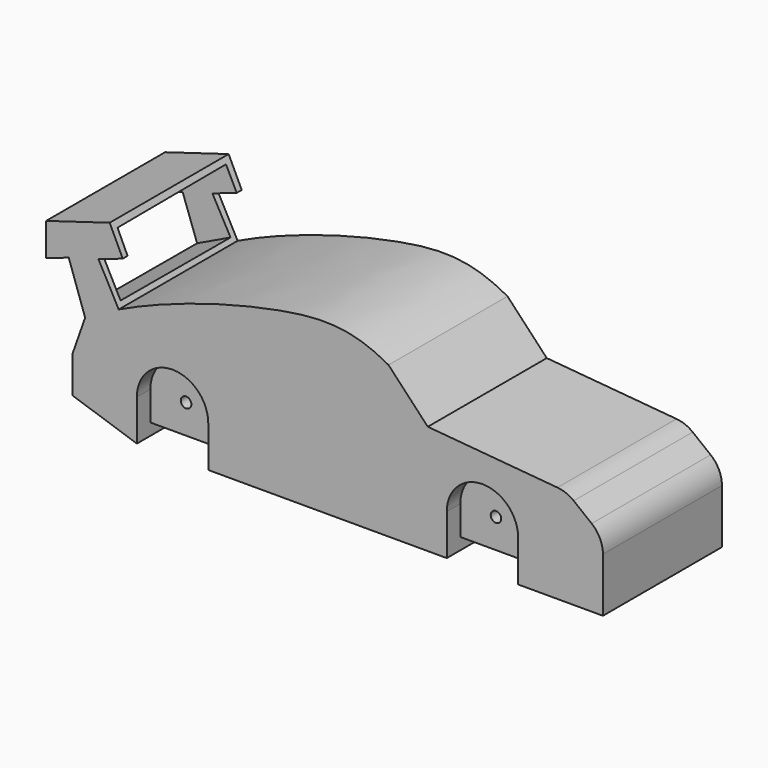
from build123d import *

# Parameters (mm, degrees)
F1_DEPTH  = 38.1
F3_DEPTH  = 25.4
F6_DEPTH  = 4.318
F8_DEPTH  = 4.318
F9_R      = 1.3609782851
F9_R_2    = 1.3503546706
F10_DEPTH = 61.214


# Not quite as in the source:
# - a feature names something its author has since deleted; it is built from what else it names


with BuildPart() as f1:
    # F0 (on Front) → F1 (new body)
    with BuildSketch(Plane.XZ):
        with BuildLine():
            Line((52.0340008008, 9.3591057662), (47.4384056476, 12.9927370075))
            ThreePointArc((47.4384056476, 12.9927370075), (45.4749605723, 14.1169814212), (43.2679541409, 14.615142718))
            Line((43.2679541409, 14.615142718), (10.0584002212, 17.5260007381))
            Line((10.0584002212, 17.5260007381), (0, 28.1940009445))
            add(Edge.make_bspline(
                [(0, 28.1940009445), (-9.1002955269, 33.2901659502), (-24.9064630473, 33.5549116559), (-55.7131559047, 24.6859865442), (-69.1292500573, 18.2258343206)],
                knots=[0, 0, 0, 0, 0.4163863711, 0.8919338321, 0.8919338321, 0.8919338321, 0.8919338321], degree=3))
            add(Edge.make_bspline(
                [(-69.1292500573, 18.2258343206), (-72.1780012369, 16.7577917973), (-75.0713687219, 15.2003305751), (-77.7240023017, 13.5635994375)],
                knots=[0.8919338321, 0.8919338321, 0.8919338321, 0.8919338321, 1, 1, 1, 1], degree=3))
            Line((-77.7240023017, 13.5635994375), (-80.9243991971, 4.4677392631))
            Line((-80.9243991971, 4.4677392631), (-80.9243991971, -5.0292001106))
            Line((-80.9243991971, -5.0292001106), (-64.465200973, -10.5156))
            Line((-64.465200973, -10.5156), (-64.465200973, -7.498764433))
            Line((-64.465200973, -7.498764433), (-64.465200973, 0))
            ThreePointArc((-64.465200973, 0), (-55.321200973, 9.144), (-46.177200973, 0))
            Line((-46.177200973, 0), (-46.177200973, -7.498764433))
            Line((-46.177200973, -7.498764433), (-46.177200973, -10.5156))
            Line((-46.177200973, -10.5156), (14.9299539626, -10.5156))
            Line((14.9299539626, -10.5156), (14.9299539626, -7.498764433))
            Line((14.9299539626, -7.498764433), (14.9299539626, 0))
            ThreePointArc((14.9299539626, 0), (24.076577276, 9.1466233134), (33.2232005894, 0))
            Line((33.2232005894, 0), (33.2232005894, -7.498764433))
            Line((33.2232005894, -7.498764433), (33.2232005894, -10.5156004429))
            Line((33.2232005894, -10.5156004429), (54.9278818071, -10.5156004429))
            Line((54.9278818071, -10.5156004429), (54.9278818071, 3.3817987423))
            ThreePointArc((54.9278818071, 3.3817987423), (54.1663592887, 6.7022936804), (52.0340008008, 9.3591057662))
        make_face()
        with BuildLine():
            add(Edge.make_bspline(
                [(-69.1292500573, 18.2258343206), (-72.1780012369, 16.7577917973), (-75.0713687219, 15.2003305751), (-77.7240023017, 13.5635994375)],
                knots=[0.8919338321, 0.8919338321, 0.8919338321, 0.8919338321, 1, 1, 1, 1], degree=3))
            Line((-69.1292500573, 18.2258343206), (-74.2949992421, 27.8891995555))
            Line((-74.2949992421, 27.8891995555), (-81.9149985909, 25.7555991411))
            Line((-81.9149985909, 25.7555991411), (-77.7240023017, 13.5635994375))
        make_face()
        with BuildLine():
            Line((14.9299539626, -7.498764433), (33.2232005894, -7.498764433))
            Line((33.2232005894, -7.498764433), (33.2232005894, 0))
            ThreePointArc((33.2232005894, 0), (24.076577276, 9.1466233134), (14.9299539626, 0))
            Line((14.9299539626, 0), (14.9299539626, -7.498764433))
        make_face()
        Polygon((-81.9149985909, 25.7555991411), (-74.2949992421, 27.8891995555), (-68.0850669491, 30.023861943), (-71.4375004172, 37.033200264), (-87.724568169, 32.1564003825), (-87.724568169, 23.7585613183), align=None)
        with BuildLine():
            Line((-64.465200973, -7.498764433), (-46.177200973, -7.498764433))
            Line((-46.177200973, -7.498764433), (-46.177200973, 0))
            ThreePointArc((-46.177200973, 0), (-55.321200973, 9.144), (-64.465200973, 0))
            Line((-64.465200973, 0), (-64.465200973, -7.498764433))
        make_face()
    extrude(amount=F1_DEPTH)

    # F2 (on face) → F3 (cut)
    with BuildSketch(Plane(origin=(-43.723380858, 0, -20.9120631104), x_dir=(0, 1, 0), z_dir=(0.9021271467, 0, 0.4314702901))):
        Polygon((-36.6774983704, 47.6490445435), (-1.5018450795, 47.5782938302), (-1.6934617888, 62.6805573702), (-36.4830493927, 62.532402575), align=None)
    extrude(amount=-F3_DEPTH, mode=Mode.SUBTRACT)

    # F5 (on face) → F6 (cut)
    with BuildSketch(Plane.XZ.offset(38.1)):
        with BuildLine():
            Line((-64.465200973, 0), (-64.465200973, -7.498764433))
            Line((-64.465200973, -7.498764433), (-46.177200973, -7.498764433))
            Line((-46.177200973, -7.498764433), (-46.177200973, 0))
            ThreePointArc((-46.177200973, 0), (-55.321200973, 9.144), (-64.465200973, 0))
        make_face()
        with BuildLine():
            Line((14.9299539626, 0), (14.9299539626, -7.498764433))
            Line((14.9299539626, -7.498764433), (33.2232005894, -7.498764433))
            Line((33.2232005894, -7.498764433), (33.2232005894, 0))
            ThreePointArc((33.2232005894, 0), (24.076577276, 9.1466233134), (14.9299539626, 0))
        make_face()
    extrude(amount=-F6_DEPTH, mode=Mode.SUBTRACT)

    # F7 (on face) → F8 (cut)
    with BuildSketch(Plane.XZ):
        with BuildLine():
            Line((14.9592272937, -8.4022274241), (33.2223922014, -8.4022274241))
            Line((33.2223922014, -8.4022274241), (33.2223922014, 0))
            ThreePointArc((33.2223922014, 0), (24.0908097476, 9.1315824538), (14.9592272937, 0))
            Line((14.9592272937, 0), (14.9592272937, -8.4022274241))
        make_face()
        with BuildLine():
            Line((-64.3822327256, -7.5330701657), (-46.1474433541, -7.5330701657))
            Line((-46.1474433541, -7.5330701657), (-46.1474433541, 0))
            ThreePointArc((-46.1474433541, 0), (-55.2648380399, 9.1173946857), (-64.3822327256, 0))
            Line((-64.3822327256, 0), (-64.3822327256, -7.5330701657))
        make_face()
    extrude(amount=F8_DEPTH, mode=Mode.SUBTRACT)

    # F9 (on face) → F10 (cut)
    with BuildSketch(Plane.XZ.offset(33.782)):
        with Locations((-55.321200973, 0)):
            Circle(F9_R)
        with Locations((24.0739539626, 0)):
            Circle(F9_R_2)
    extrude(amount=-F10_DEPTH, mode=Mode.SUBTRACT)


solid = f1.part
